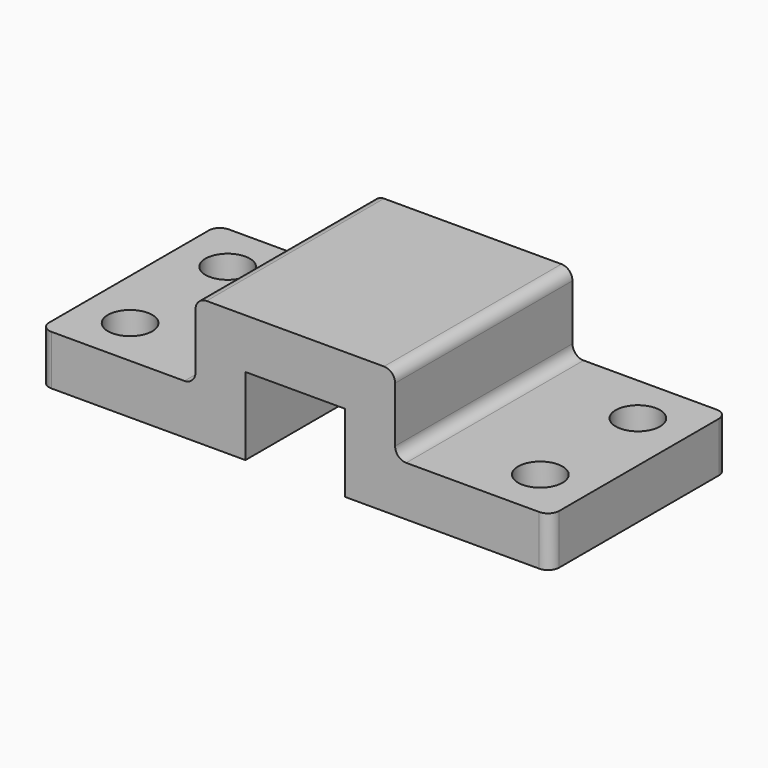
from build123d import *

# Parameters (mm, degrees)
F1_DEPTH = 1016
F2_R     = 50.8
F3_R     = 50.8
F4_R     = 101.6
F5_DEPTH = 228.6


# Not quite as in the source:
# - a feature names something its author has since deleted; it is built from what else it names


with BuildPart() as f1:
    # F0 (on Front) → F1 (new body)
    with BuildSketch(Plane.XZ):
        Polygon((-1270.8357659235, 228.6), (-1270.8357659235, 0), (-331.0357659235, 0), (-331.0357659235, 355.6), (126.1642340765, 355.6), (126.1642340765, 0), (1065.9642340765, 0), (1065.9642340765, 228.6), (354.7642340765, 228.6), (354.7642340765, 584.2), (-559.6357659235, 584.2), (-559.6357659235, 228.6), align=None)
    extrude(amount=F1_DEPTH)

    # F2
    f2_edges = [f1.edges().sort_by_distance(p)[0] for p in [
        (-559.635766, -508, 584.2),
        (354.764234, -508, 584.2),
        (-1270.835766, -1016, 114.3),
        (1065.964234, -1016, 114.3),
        (1065.964234, 0, 114.3),
        (-1270.835766, 0, 114.3),
    ]]
    fillet(f2_edges, radius=F2_R)

    # F3
    f3_edges = [f1.edges().sort_by_distance(p)[0] for p in [
        (354.764234, -508, 228.6),
        (-559.635766, -508, 228.6),
    ]]
    fillet(f3_edges, radius=F3_R)

    # F4 (on face) → F5 (cut)
    with BuildSketch(Plane(origin=(0, 0, 0), x_dir=(1, 0, 0), z_dir=(0, 0, -1))):
        with Locations((837.3642340765, 228.6)):
            Circle(F4_R)
        with Locations((837.3642340765, 787.4)):
            Circle(F4_R)
        with Locations((-1042.2357659235, 228.6)):
            Circle(F4_R)
        with Locations((-1042.2357659235, 787.4)):
            Circle(F4_R)
    extrude(amount=-F5_DEPTH, mode=Mode.SUBTRACT)


solid = f1.part
